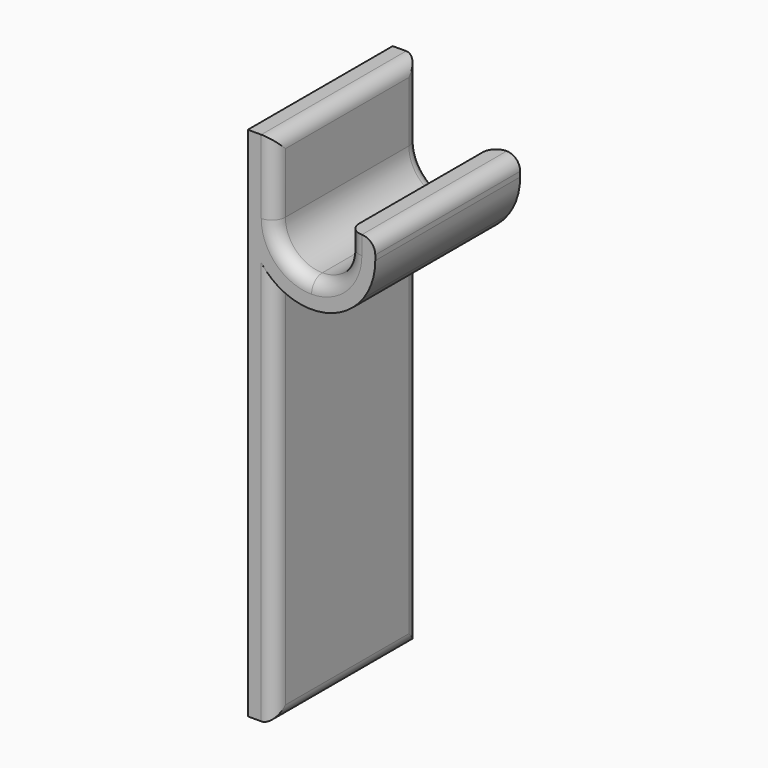
from build123d import *

# Parameters (mm, degrees)
F1_W     = 4
F1_H     = 2.75
F2_DEPTH = 27
F3_R     = 1.99999


# Not quite as in the source:
# - a fillet or chamfer is up to 0.001 mm smaller than in the source, because OpenCascade refuses the exact size


with BuildPart() as f2:
    # F1 (on Front) → F2 (new body)
    with BuildSketch(Plane.XZ):
        with BuildLine():
            Line((4, 16.5), (0, 16.5))
            Line((0, 16.5), (0, 5.5))
            ThreePointArc((0, 5.5), (1.0590284919, 9.8588989435), (4, 13.2459666924))
            Line((4, 13.2459666924), (4, 16.5))
        make_face()
        with BuildLine():
            ThreePointArc((1.7540333076, 0), (0.4491248054, 2.6135388083), (0, 5.5))
            Line((0, 5.5), (0, 0))
            Line((0, 0), (1.7540333076, 0))
        make_face()
        with BuildLine():
            Line((4, 5.5), (0, 5.5))
            ThreePointArc((0, 5.5), (0.4491248054, 2.6135388083), (1.7540333076, 0))
            Line((1.7540333076, 0), (4, 0))
            Line((4, 0), (4, 5.5))
        make_face()
        with BuildLine():
            ThreePointArc((4, 13.2459666924), (1.0590284919, 9.8588989435), (0, 5.5))
            Line((0, 5.5), (4, 5.5))
            Line((4, 5.5), (4, 13.2459666924))
        make_face()
        with BuildLine():
            Line((1.7540333076, 0), (0, 0))
            Line((0, 0), (0, -60.5))
            Line((0, -60.5), (4, -60.5))
            Line((4, -60.5), (4, -2.2459666924))
            ThreePointArc((4, -2.2459666924), (2.7824855787, -1.2175144213), (1.7540333076, 0))
        make_face()
        with BuildLine():
            Line((4, 0), (1.7540333076, 0))
            ThreePointArc((1.7540333076, 0), (2.7824855787, -1.2175144213), (4, -2.2459666924))
            Line((4, -2.2459666924), (4, 0))
        make_face()
        with BuildLine():
            ThreePointArc((9.5, 0), (5.6109127035, 1.6109127035), (4, 5.5))
            Line((4, 5.5), (4, 0))
            Line((4, 0), (9.5, 0))
        make_face()
        with BuildLine():
            Line((9.5, 0), (4, 0))
            Line((4, 0), (4, -2.2459666924))
            ThreePointArc((4, -2.2459666924), (11.0881382785, -3.8663128716), (17.2459666924, 0))
            Line((17.2459666924, 0), (9.5, 0))
        make_face()
        with BuildLine():
            ThreePointArc((15, 5.5), (13.3890872965, 1.6109127035), (9.5, 0))
            Line((9.5, 0), (17.2459666924, 0))
            ThreePointArc((17.2459666924, 0), (18.5508751946, 2.6135388083), (19, 5.5))
            Line((19, 5.5), (15, 5.5))
        make_face()
        with Locations((17, 6.875)):
            Rectangle(F1_W, F1_H)
    extrude(amount=F2_DEPTH)

    # F3 (radius 2 in the source; OpenCascade refuses exactly that, so slightly less here)
    f3_edges = [f2.edges().sort_by_distance(p)[0] for p in [
        (4, -27, -31.372983),
        (4, -27, 11),
        (4, 0, -31.372983),
        (4, -13.5, -60.5),
        (4, 0, 11),
        (19, -13.5, 8.25),
        (4, -13.5, 16.5),
    ]]
    fillet(f3_edges, radius=F3_R)


solid = f2.part
